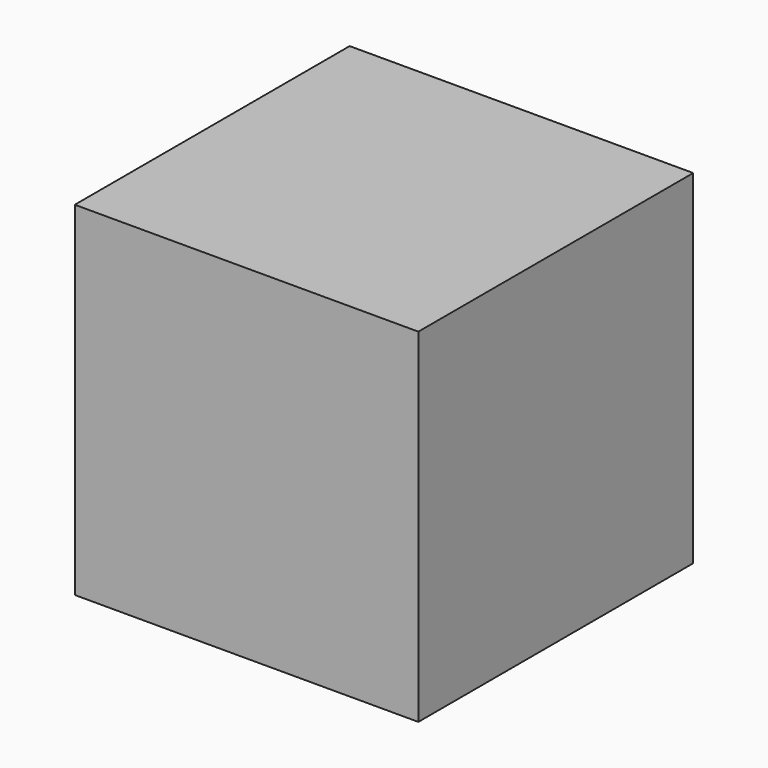
from build123d import *

# Parameters (mm, degrees)
F0_W      = 165.1
F0_H      = 165.1
F1_DEPTH  = 2.3622
F2_W      = 2.3622
F2_H      = 165.1
F2_W_2    = 162.7378
F3_DEPTH  = 2.3622
F4_W      = 162.7378
F4_H      = 165.1
F4_W_2    = 2.3622
F5_DEPTH  = 2.3622
F6_W      = 162.7378
F6_H      = 165.1
F6_W_2    = 2.3622
F7_DEPTH  = 2.3622
F8_W      = 167.4622
F8_H      = 167.4622
F8_W_2    = 162.7378
F8_H_2    = 162.7378
F9_DEPTH  = 2.3622
F10_W     = 25.4
F10_H     = 25.4
F10_H_2   = 2.3622
F10_W_2   = 2.3622
F11_DEPTH = 2.3622


with BuildPart() as f1:
    # F0 (on Front) → F1 (new body)
    with BuildSketch(Plane.XZ):
        with Locations((82.55, 82.55)):
            Rectangle(F0_W, F0_H)
    extrude(amount=F1_DEPTH)

    # F2 (on face) → F3 (join)
    with BuildSketch(Plane.YZ.offset(165.1)):
        with Locations((-1.1811, 82.55)):
            Rectangle(F2_W, F2_H)
        with Locations((81.3689, 82.55)):
            Rectangle(F2_W_2, F2_H)
    extrude(amount=F3_DEPTH)

    # F4 (on face) → F5 (join)
    with BuildSketch(Plane(origin=(0, 162.7378, 0), x_dir=(-1, 0, 0), z_dir=(0, 1, 0))):
        with Locations((-83.7311, 82.55)):
            Rectangle(F4_W, F4_H)
        with Locations((-166.2811, 82.55)):
            Rectangle(F4_W_2, F4_H)
    extrude(amount=F5_DEPTH)

    # F6 (on face) → F7 (join)
    with BuildSketch(Plane(origin=(2.3622, 0, 0), x_dir=(0, -1, 0), z_dir=(-1, 0, 0))):
        with Locations((-81.3689, 82.55)):
            Rectangle(F6_W, F6_H)
        with Locations((-163.9189, 82.55)):
            Rectangle(F6_W_2, F6_H)
    extrude(amount=F7_DEPTH)

    # F8 (on face) → F9 (join)
    with BuildSketch(Plane.XY.offset(165.1)):
        with Locations((83.7311, 81.3689)):
            Rectangle(F8_W, F8_H)
        with Locations((83.7311, 81.3689)):
            Rectangle(F8_W_2, F8_H_2, mode=Mode.SUBTRACT)
        with Locations((83.7311, 81.3689)):
            Rectangle(F8_W_2, F8_H_2)
    extrude(amount=F9_DEPTH)

    # F10 (on face) → F11 (join)
    with BuildSketch(Plane(origin=(0, 0, 0), x_dir=(1, 0, 0), z_dir=(0, 0, -1))):
        with Locations((127, -12.7)):
            Rectangle(F10_W, F10_H)
        with Locations((152.4, -124.6378)):
            Rectangle(F10_W, F10_H)
        with Locations((40.4622, -12.7)):
            Rectangle(F10_W, F10_H)
        with Locations((15.0622, -124.6378)):
            Rectangle(F10_W, F10_H)
        with Locations((40.4622, 1.1811)):
            Rectangle(F10_W, F10_H_2)
        with Locations((127, 1.1811)):
            Rectangle(F10_W, F10_H_2)
        with Locations((1.1811, -124.6378)):
            Rectangle(F10_W_2, F10_H)
        with Locations((166.2811, -124.6378)):
            Rectangle(F10_W_2, F10_H)
    extrude(amount=-F11_DEPTH)


solid = f1.part
